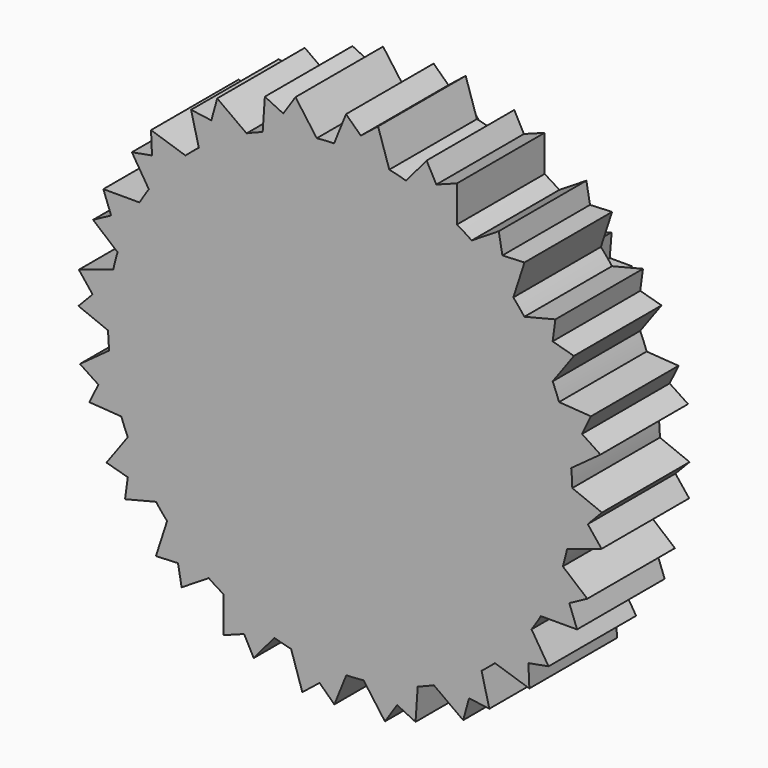
from build123d import *

# Parameters (mm, degrees)
F0_R            = 53.8517918496
F1_DEPTH        = 12.7
F3_DEPTH        = 25.4
F3_COPIES_COUNT = 20
F5_DEPTH        = 12.7
F5_COPIES_COUNT = 8
F7_DEPTH        = 12.7
F7_COPIES_COUNT = 4


# Not quite as in the source:
# - a pattern or mirror of a feature is missing from the dataset's text; its kind, count and spacing are read off the source's solid


with BuildPart() as f1:
    # F0 (on Front) → F1 (new body, symmetric)
    with BuildSketch(Plane.XZ):
        Circle(F0_R)
    extrude(amount=F1_DEPTH, both=True)

    # F2 (on face) → F3 (join, through all)
    with BuildSketch(Plane.XZ.offset(12.7)):
        Polygon((17.4729507416, -58.154836297), (17.9823680134, -50.7607124264), (5.4343099044, -53.5768957786), (10.3754857555, -60.3680238128), (13.1992083043, -56.0942813754), align=None)
    f3 = extrude(amount=-F3_DEPTH)

    # F3_copies: F3 ×20 about axis
    f3_copies_axis = Axis((0, 0, 0), (0, 1, 0))
    for i in range(1, F3_COPIES_COUNT):
        add(f3.rotate(f3_copies_axis, i * 360 / F3_COPIES_COUNT))

    # F4 (on face) → F5 (join)
    with BuildSketch(Plane(origin=(0, 12.7, 0), x_dir=(-1, 0, 0), z_dir=(0, 1, 0))):
        Polygon((32.4746519327, -31.217938289), (32.0429392159, -25.8215237409), (37.223495543, -25.8215237409), (32.9063646495, -20.5330364406), (25.2434555441, -28.7355873734), align=None)
    f5 = extrude(amount=F5_DEPTH)

    # F5_copies: F5 ×8 about axis
    f5_copies_axis = Axis((0, 0, 0), (0, 1, 0))
    for i in range(1, F5_COPIES_COUNT):
        add(f5.rotate(f5_copies_axis, i * 360 / F5_COPIES_COUNT))

    # F6 (on face) → F7 (join)
    with BuildSketch(Plane(origin=(0, 12.7, 0), x_dir=(-1, 0, 0), z_dir=(0, 1, 0))):
        Polygon((-18.7933090678, 14.4219585457), (-26.7386548221, 15.6052242965), (-29.1993897408, 5.2935681306), (-20.8797585219, 5.2935681306), (-24.5122741908, 10.0978622213), align=None)
    f7 = extrude(amount=F7_DEPTH)

    # F7_copies: F7 ×4 about axis
    f7_copies_axis = Axis((0, 0, 0), (0, 1, 0))
    for i in range(1, F7_COPIES_COUNT):
        add(f7.rotate(f7_copies_axis, i * 360 / F7_COPIES_COUNT))


solid = f1.part
